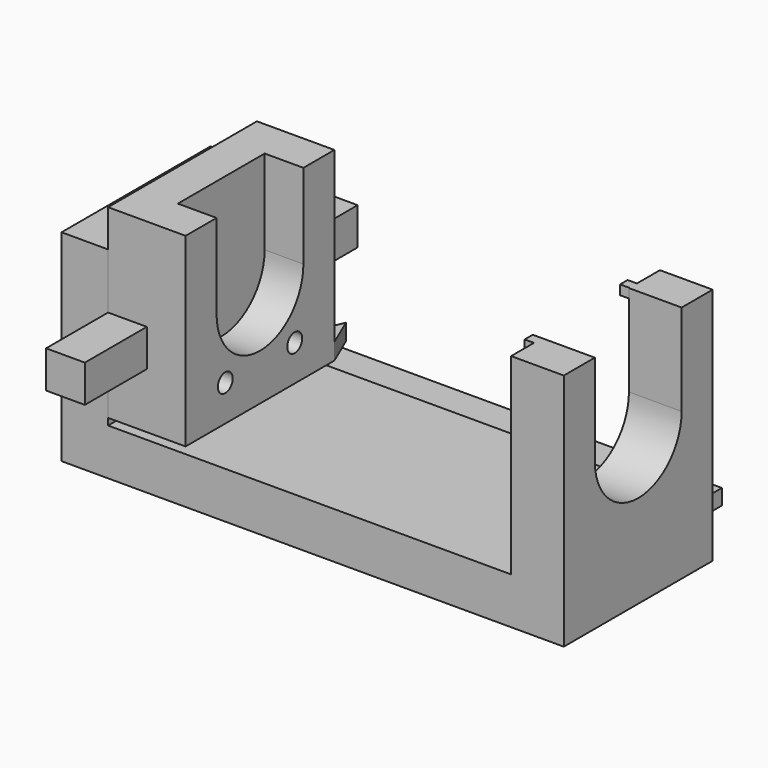
from build123d import *

# Parameters (mm, degrees)
F0_W      = 15
F0_H      = 60
F1_DEPTH  = 65
F0_W_2    = 17
F0_W_3    = 130
F2_DEPTH  = 15
F4_DEPTH  = 17
F5_R      = 3
F6_DEPTH  = 155
F7_W      = 60
F7_H      = 49.8176734522
F7_R      = 3
F8_DEPTH  = 25
F10_DEPTH = 12.5
F12_W     = 25
F12_H     = 60
F13_DEPTH = 2
F15_DEPTH = 25
F16_W     = 12.5
F16_H     = 12
F17_DEPTH = 25
F18_DEPTH = 25
F19_W     = 12.5
F19_H     = 12
F20_DEPTH = 25
F21_DEPTH = 12
F22_W     = 8.5935546458
F22_H     = 5.2922566906
F23_DEPTH = 10
F25_DEPTH = 10
F26_DEPTH = 12
F27_W     = 3.2838956267
F27_H     = 3.0892942548
F27_W_2   = 3.0268859118
F28_DEPTH = 3


# Not quite as in the source:
# - a feature names something its author has since deleted; it is built from what else it names


with BuildPart() as f1:
    # F0 (on Top) → F1 (new body)
    with BuildSketch(Plane.XY):
        with Locations((-72.5, 0)):
            Rectangle(F0_W, F0_H)
    extrude(amount=F1_DEPTH)



with BuildPart() as f1b:
    # F0 (on Top) → F1, piece 2 (new body)
    with BuildSketch(Plane.XY):
        with Locations((73.5, 0)):
            Rectangle(F0_W_2, F0_H)
    extrude(amount=F1_DEPTH)


with BuildPart() as f1_1:
    add(f1.part)

    add(f1b.part)  # F2 merges F1b
    # F0 (on Top) → F2 (join)
    with BuildSketch(Plane.XY):
        Rectangle(F0_W_3, F0_H)
    extrude(amount=F2_DEPTH)

    # F3 (on face) → F4 (cut)
    with BuildSketch(Plane.YZ.offset(82)):
        with BuildLine():
            ThreePointArc((-17.5, 47.5), (0, 30), (17.5, 47.5))
            ThreePointArc((17.5, 47.5), (0, 65), (-17.5, 47.5))
        make_face()
        with BuildLine():
            Line((-17.5, 65), (-17.5, 47.5))
            ThreePointArc((-17.5, 47.5), (-12.3743686586, 59.8743686829), (3.43e-08, 65))
            Line((3.43e-08, 65), (-17.5, 65))
        make_face()
        with BuildLine():
            ThreePointArc((3.43e-08, 65), (12.3743686829, 59.8743686586), (17.5, 47.5))
            Line((17.5, 47.5), (17.5, 65))
            Line((17.5, 65), (3.43e-08, 65))
        make_face()
    extrude(amount=-F4_DEPTH, mode=Mode.SUBTRACT)

    # F5 (on face) → F6 (cut)
    with BuildSketch(Plane(origin=(-80, 0, 0), x_dir=(0, -1, 0), z_dir=(-1, 0, 0))):
        with Locations((-14, 28.7966762781)):
            Circle(F5_R)
        with Locations((14, 28.7966762781)):
            Circle(F5_R)
    extrude(amount=-F6_DEPTH, mode=Mode.SUBTRACT)

    # F11: union 

    # F14 (on face) → F15 (join)
    with BuildSketch(Plane(origin=(0, 30, 0), x_dir=(-1, 0, 0), z_dir=(0, 1, 0))):
        Polygon((-65, 4.9993242615), (-65, 0), (65, 0), (64.9177994628, 4.9993242615), align=None)
    extrude(amount=F15_DEPTH)

    # F26 (add): faces of the model
    f26_faces = [f1_1.faces().sort_by_distance(p)[0] for p in [
        (73.5, -23.75, 65),
        (73.5, 23.75, 65),
    ]]
    extrude(f26_faces, amount=F26_DEPTH)

    # F27 (on face) → F28 (join)
    with BuildSketch(Plane(origin=(65, 0, 0), x_dir=(0, -1, 0), z_dir=(-1, 0, 0))):
        with Locations((19.1419478133, 75.4553528726)):
            Rectangle(F27_W, F27_H)
        with Locations((-19.2088121548, 75.4553528726)):
            Rectangle(F27_W_2, F27_H)
    extrude(amount=F28_DEPTH)


with BuildPart() as f8:
    # F7 (on face) → F8 (new body)
    with BuildSketch(Plane.YZ.offset(-65)):
        with Locations((0, 40.0911632739)):
            Rectangle(F7_W, F7_H)
        with Locations((-14, 28.7966762781)):
            Circle(F7_R, mode=Mode.SUBTRACT)
        with Locations((14, 28.7966762781)):
            Circle(F7_R, mode=Mode.SUBTRACT)
    extrude(amount=F8_DEPTH)

    # F9 (on face) → F10 (cut)
    with BuildSketch(Plane.YZ.offset(-40)):
        with BuildLine():
            ThreePointArc((-17.5, 49.6503765881), (0, 32.1503765881), (17.5, 49.6503765881))
            ThreePointArc((17.5, 49.6503765881), (15.0554364312, 58.5713537692), (8.4047047011, 65))
            Line((8.4047047011, 65), (-8.4047047011, 65))
            ThreePointArc((-8.4047047011, 65), (-15.0554364312, 58.5713537692), (-17.5, 49.6503765881))
        make_face()
        with BuildLine():
            ThreePointArc((8.4047047011, 65), (15.0554364312, 58.5713537692), (17.5, 49.6503765881))
            Line((17.5, 49.6503765881), (17.5, 65))
            Line((17.5, 65), (8.4047047011, 65))
        make_face()
        with BuildLine():
            Line((-17.5, 65), (-17.5, 49.6503765881))
            ThreePointArc((-17.5, 49.6503765881), (-15.0554364312, 58.5713537692), (-8.4047047011, 65))
            Line((-8.4047047011, 65), (-17.5, 65))
        make_face()
    extrude(amount=-F10_DEPTH, mode=Mode.SUBTRACT)

    # F12 (on face) → F13 (cut)
    with BuildSketch(Plane(origin=(0, 0, 15.1823265478), x_dir=(1, 0, 0), z_dir=(0, 0, -1))):
        with Locations((-52.5, 0)):
            Rectangle(F12_W, F12_H)
    extrude(amount=-F13_DEPTH, mode=Mode.SUBTRACT)

    # F16 (on face) → F17 (join)
    with BuildSketch(Plane.XZ.offset(30)):
        with Locations((-58.75, 41.0911632739)):
            Rectangle(F16_W, F16_H)
    extrude(amount=F17_DEPTH)

    # F19 (on face) → F20 (join)
    with BuildSketch(Plane(origin=(0, 30, 0), x_dir=(-1, 0, 0), z_dir=(0, 1, 0))):
        with Locations((58.75, 41.0911632739)):
            Rectangle(F19_W, F19_H)
    extrude(amount=F20_DEPTH)

    # F21 (add): a face of the model
    f21_faces = [f8.faces().sort_by_distance(p)[0] for p in [
        (-55.0735294118, 0, 65),
    ]]
    extrude(f21_faces, amount=F21_DEPTH)

    # F22 (on face) → F23 (join)
    with BuildSketch(Plane(origin=(0, 30, 0), x_dir=(-1, 0, 0), z_dir=(0, 1, 0))):
        with Locations((44.2967773229, 19.8284548931)):
            Rectangle(F22_W, F22_H)
    extrude(amount=F23_DEPTH)

    # F24 (on face) → F25 (cut)
    with BuildSketch(Plane.XY.offset(22.4745832384)):
        Polygon((-44.2967773229, 40), (-40, 30), (-40, 40), align=None)
        Polygon((-48.5935546458, 30), (-44.2967773229, 40), (-48.5935546458, 40), align=None)
    extrude(amount=-F25_DEPTH, mode=Mode.SUBTRACT)


with BuildPart() as f18:
    # F16 (on face) → F18 (new body)
    with BuildSketch(Plane.XZ.offset(30)):
        with Locations((-58.75, 41.0911632739)):
            Rectangle(F16_W, F16_H)
    extrude(amount=F18_DEPTH)


solid = Compound([f1_1.part, f8.part])
